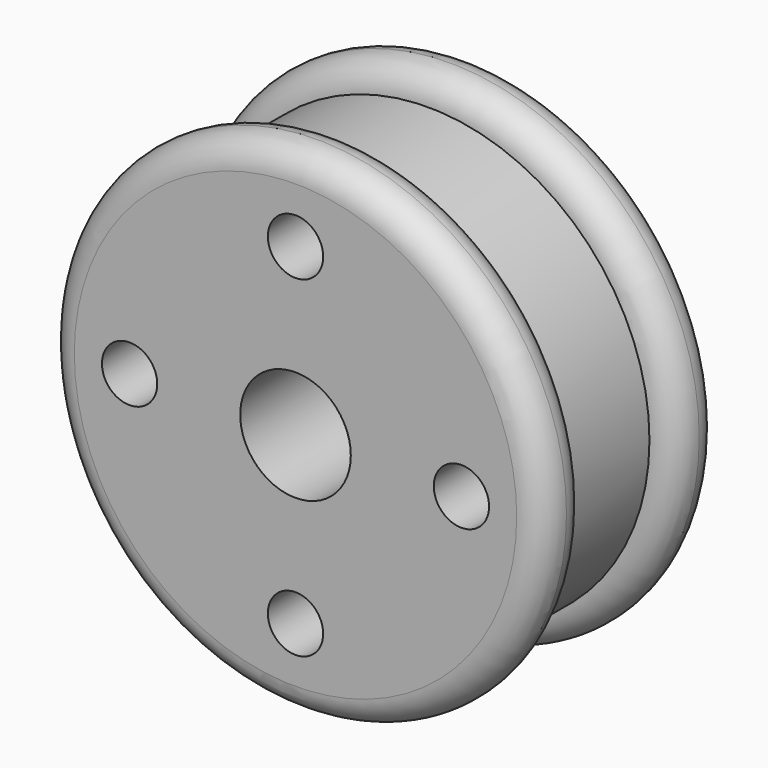
from build123d import *

# Parameters (mm, degrees)
F0_R     = 28.575
F1_DEPTH = 6.35
F2_R     = 3.17499
F3_R     = 25.4
F4_DEPTH = 12.7
F5_R     = 28.575
F6_DEPTH = 6.35
F7_R     = 3.17499
F8_R     = 6.35
F8_R_2   = 3.175
F9_DEPTH = 25.401


# Not quite as in the source:
# - a fillet or chamfer is up to 0.001 mm smaller than in the source, because OpenCascade refuses the exact size


with BuildPart() as f1:
    # F0 (on Front) → F1 (new body)
    with BuildSketch(Plane.XZ):
        Circle(F0_R)
    extrude(amount=F1_DEPTH)

    # F2 (radius 3.175 in the source; OpenCascade refuses exactly that, so slightly less here)
    f2_edges = [f1.edges().sort_by_distance(p)[0] for p in [
        (28.575, -3.175, 0),
        (-28.575, 0, 0),
        (-28.575, -6.35, 0),
    ]]
    fillet(f2_edges, radius=F2_R)

    # F3 (on face) → F4 (join)
    with BuildSketch(Plane.XZ.offset(6.35)):
        Circle(F3_R)
    extrude(amount=F4_DEPTH)

    # F5 (on face) → F6 (join)
    with BuildSketch(Plane.XZ.offset(19.05)):
        Circle(F5_R)
    extrude(amount=F6_DEPTH)

    # F7 (radius 3.175 in the source; OpenCascade refuses exactly that, so slightly less here)
    f7_edges = [f1.edges().sort_by_distance(p)[0] for p in [
        (28.575, -22.225, 0),
        (-28.575, -19.05, 0),
        (-28.575, -25.4, 0),
    ]]
    fillet(f7_edges, radius=F7_R)

    # F8 (on face) → F9 (cut, through all)
    with BuildSketch(Plane.XZ.offset(25.4)):
        Circle(F8_R)
        with Locations((0, 19.05)):
            Circle(F8_R_2)
        with Locations((-19.05, 0)):
            Circle(F8_R_2)
        with Locations((19.05, 0)):
            Circle(F8_R_2)
        with Locations((0, -19.05)):
            Circle(F8_R_2)
    extrude(amount=-F9_DEPTH, mode=Mode.SUBTRACT)


solid = f1.part
